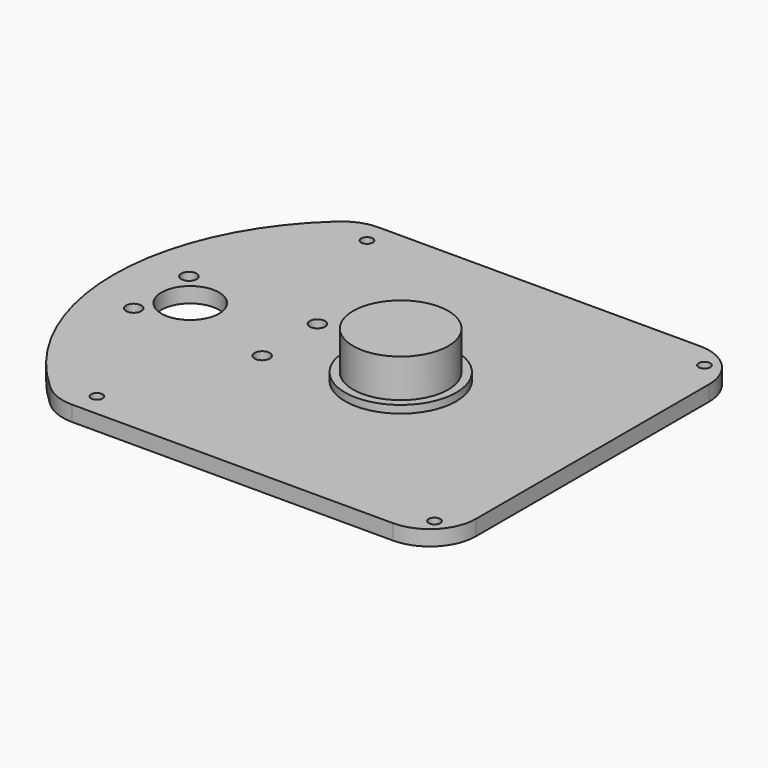
from build123d import *

# Parameters (mm, degrees)
F0_R     = 1.5
F0_R_2   = 2
F0_R_3   = 14.5
F1_DEPTH = 4
F2_R     = 12
F0_R_4   = 12.4
F3_DEPTH = 6
F4_DEPTH = 16


with BuildPart() as f1:
    # F0 (on Top) → F1 (new body)
    with BuildSketch(Plane.XY):
        with BuildLine():
            Line((40.1261364576, -50), (50, -50))
            Line((50, -50), (50, -40.1261364576))
            ThreePointArc((50, -40.1261364576), (48.5323223277, -39.658202653), (47, -39.5))
            Line((47, -39.5), (47, -47))
            Line((47, -47), (39.5, -47))
            ThreePointArc((39.5, -47), (39.658202653, -48.5323223277), (40.1261364576, -50))
        make_face()
        with BuildLine():
            Line((-40.1261364576, -50), (40.1261364576, -50))
            ThreePointArc((40.1261364576, -50), (39.658202653, -48.5323223277), (39.5, -47))
            Line((39.5, -47), (-39.5, -47))
            ThreePointArc((-39.5, -47), (-39.658202653, -48.5323223277), (-40.1261364576, -50))
        make_face()
        with BuildLine():
            ThreePointArc((47, -39.5), (48.5323223277, -39.658202653), (50, -40.1261364576))
            Line((50, -40.1261364576), (50, 40.1261364576))
            ThreePointArc((50, 40.1261364576), (48.5323223277, 39.658202653), (47, 39.5))
            Line((47, 39.5), (47, -39.5))
        make_face()
        with BuildLine():
            Line((-50, -50), (-40.1261364576, -50))
            ThreePointArc((-40.1261364576, -50), (-39.658202653, -48.5323223277), (-39.5, -47))
            Line((-39.5, -47), (-47, -47))
            Line((-47, -47), (-47, -39.5))
            ThreePointArc((-47, -39.5), (-52.0432569895, -41.4488236438), (-54.4656023889, -46.2825176166))
            ThreePointArc((-54.4656023889, -46.2825176166), (-52.2758824324, -48.1930098751), (-50, -50))
        make_face()
        with BuildLine():
            ThreePointArc((47, -39.5), (41.6966991411, -41.6966991411), (39.5, -47))
            Line((39.5, -47), (47, -47))
            Line((47, -47), (47, -39.5))
        make_face()
        with Locations((44, -44)):
            Circle(F0_R, mode=Mode.SUBTRACT)
        with BuildLine():
            Line((-39.5, -47), (39.5, -47))
            ThreePointArc((39.5, -47), (41.6966991411, -41.6966991411), (47, -39.5))
            Line((47, -39.5), (47, 39.5))
            ThreePointArc((47, 39.5), (41.6966991411, 41.6966991411), (39.5, 47))
            Line((39.5, 47), (-39.5, 47))
            ThreePointArc((-39.5, 47), (-41.6966991411, 41.6966991411), (-47, 39.5))
            Line((-47, 39.5), (-47, -39.5))
            ThreePointArc((-47, -39.5), (-41.6966991411, -41.6966991411), (-39.5, -47))
        make_face()
        with Locations((-28.9172229711, -9)):
            Circle(F0_R_2, mode=Mode.SUBTRACT)
        with Locations((-28.9172229711, 9)):
            Circle(F0_R_2, mode=Mode.SUBTRACT)
        Circle(F0_R_3, mode=Mode.SUBTRACT)
        with BuildLine():
            ThreePointArc((47, 39.5), (48.5323223277, 39.658202653), (50, 40.1261364576))
            Line((50, 40.1261364576), (50, 50))
            Line((50, 50), (40.1261364576, 50))
            ThreePointArc((40.1261364576, 50), (39.658202653, 48.5323223277), (39.5, 47))
            Line((39.5, 47), (47, 47))
            Line((47, 47), (47, 39.5))
        make_face()
        with BuildLine():
            ThreePointArc((-74.8632505062, 0), (-69.5376936802, -25.2890069281), (-54.4656023889, -46.2825176166))
            ThreePointArc((-54.4656023889, -46.2825176166), (-52.0432569895, -41.4488236438), (-47, -39.5))
            Line((-47, -39.5), (-47, 39.5))
            ThreePointArc((-47, 39.5), (-52.0432569895, 41.4488236438), (-54.4656023889, 46.2825176166))
            ThreePointArc((-54.4656023889, 46.2825176166), (-69.5376936802, 25.2890069281), (-74.8632505062, 0))
        make_face()
        with Locations((-62.4172229711, -9)):
            Circle(F0_R_2, mode=Mode.SUBTRACT)
        with Locations((-62.4172229711, 9)):
            Circle(F0_R_2, mode=Mode.SUBTRACT)
        with BuildLine():
            ThreePointArc((-47.3632505062, 0), (-54.8632505062, -7.5), (-62.3632505062, 0))
            ThreePointArc((-62.3632505062, 0), (-54.8632505062, 7.5), (-47.3632505062, 0))
        make_face(mode=Mode.SUBTRACT)
        with BuildLine():
            Line((-47, -47), (-39.5, -47))
            ThreePointArc((-39.5, -47), (-41.6966991411, -41.6966991411), (-47, -39.5))
            Line((-47, -39.5), (-47, -47))
        make_face()
        with Locations((-44, -44)):
            Circle(F0_R, mode=Mode.SUBTRACT)
        with BuildLine():
            ThreePointArc((39.5, 47), (41.6966991411, 41.6966991411), (47, 39.5))
            Line((47, 39.5), (47, 47))
            Line((47, 47), (39.5, 47))
        make_face()
        with Locations((44, 44)):
            Circle(F0_R, mode=Mode.SUBTRACT)
        with BuildLine():
            ThreePointArc((39.5, 47), (39.658202653, 48.5323223277), (40.1261364576, 50))
            Line((40.1261364576, 50), (-40.1261364576, 50))
            ThreePointArc((-40.1261364576, 50), (-39.658202653, 48.5323223277), (-39.5, 47))
            Line((-39.5, 47), (39.5, 47))
        make_face()
        with BuildLine():
            ThreePointArc((-54.4656023889, 46.2825176166), (-52.0432569895, 41.4488236438), (-47, 39.5))
            Line((-47, 39.5), (-47, 47))
            Line((-47, 47), (-39.5, 47))
            ThreePointArc((-39.5, 47), (-39.658202653, 48.5323223277), (-40.1261364576, 50))
            Line((-40.1261364576, 50), (-50, 50))
            ThreePointArc((-50, 50), (-52.2758824324, 48.1930098751), (-54.4656023889, 46.2825176166))
        make_face()
        with BuildLine():
            Line((-47, 47), (-47, 39.5))
            ThreePointArc((-47, 39.5), (-41.6966991411, 41.6966991411), (-39.5, 47))
            Line((-39.5, 47), (-47, 47))
        make_face()
        with Locations((-44, 44)):
            Circle(F0_R, mode=Mode.SUBTRACT)
    extrude(amount=F1_DEPTH)

    # F2
    f2_edges = [f1.edges().sort_by_distance(p)[0] for p in [
        (-50, 50, 2),
        (50, 50, 2),
        (50, -50, 2),
        (-50, -50, 2),
    ]]
    fillet(f2_edges, radius=F2_R)

    # F0 (on Top) → F3 (join)
    with BuildSketch(Plane.XY):
        Circle(F0_R_3)
        Circle(F0_R_4, mode=Mode.SUBTRACT)
    extrude(amount=F3_DEPTH)

    # F0 (on Top) → F4 (join)
    with BuildSketch(Plane.XY):
        Circle(F0_R_4)
    extrude(amount=F4_DEPTH)


solid = f1.part
